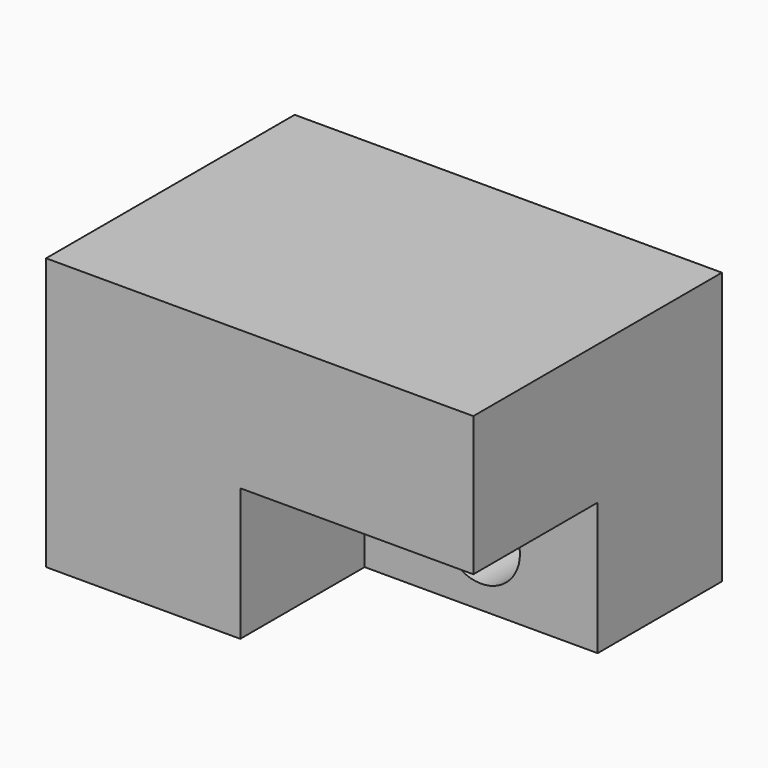
from build123d import *

# Parameters (mm, degrees)
F0_W     = 55
F0_H     = 35
F1_DEPTH = 40
F2_W     = 30
F2_H     = 17.0720907301
F3_DEPTH = 20
F4_R     = 5
F5_DEPTH = 40.001


# Not quite as in the source:
# - a feature names something its author has since deleted; it is built from what else it names


with BuildPart() as f1:
    # F0 (on Front) → F1 (new body)
    with BuildSketch(Plane.XZ):
        with Locations((27.5, -17.5)):
            Rectangle(F0_W, F0_H)
    extrude(amount=F1_DEPTH)

    # F2 (on face) → F3 (cut)
    with BuildSketch(Plane.XZ.offset(40)):
        with Locations((40, -26.463954635)):
            Rectangle(F2_W, F2_H)
    extrude(amount=-F3_DEPTH, mode=Mode.SUBTRACT)

    # F4 (on Front) → F5 (cut, through all)
    with BuildSketch(Plane.XZ):
        with Locations((40, -27)):
            Circle(F4_R)
    extrude(amount=F5_DEPTH, mode=Mode.SUBTRACT)


solid = f1.part
